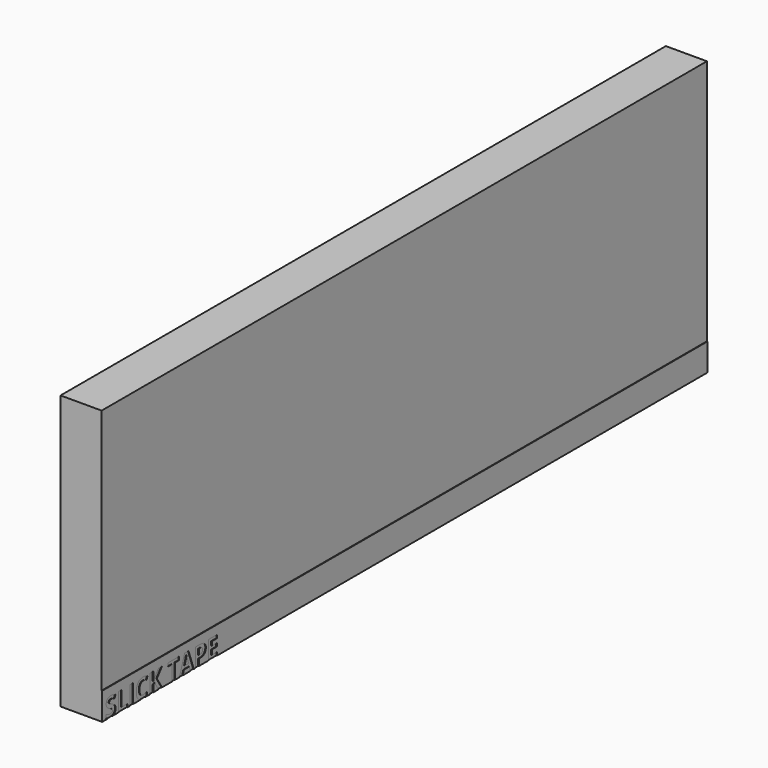
from build123d import *

# Parameters (mm, degrees)
F1_DEPTH     = 175.41875
F3_TEXT_SIZE = 12.0244892107
F4_DEPTH     = 0.254


# Not quite as in the source:
# - Text() gives the source's letters only with a copy of the font that has no kerning and outlines rounded to 1/6400 em; it was checked with that copy


with BuildPart() as f1:
    # F0 (on Front) → F1 (new body, symmetric)
    with BuildSketch(Plane.XZ):
        Polygon((9.525, 63.5), (-9.525, 63.5), (-9.525, -63.5), (9.779, -63.5), (9.779, -50.8), (9.525, -50.8), (9.525, 50.8), align=None)
    extrude(amount=F1_DEPTH, both=True)

    # F3 (on face) → F4 (cut)
    with BuildSketch(Plane.YZ.offset(9.779)):
        with Locations((-173.7722158432, -63.5)):
            Text('SLICK TAPE', F3_TEXT_SIZE, font='Open Sans', font_style=FontStyle.BOLD, text_align=(TextAlign.LEFT, TextAlign.BOTTOM))
    extrude(amount=-F4_DEPTH, mode=Mode.SUBTRACT)


solid = f1.part
